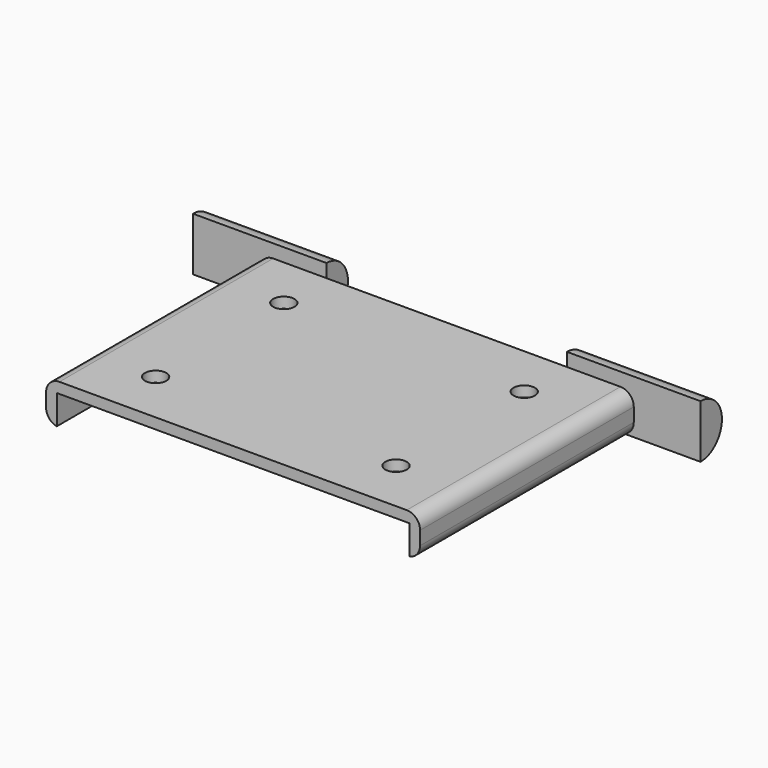
from build123d import *

# Parameters (mm, degrees)
F1_DEPTH    = 100
F2_T1_DEPTH = 125
F2_T3_DEPTH = 124.4948974279
F3_T1_DEPTH = 124.4948974279
F3_T3_DEPTH = 125
F5_D        = 8
F7_R        = 7.5
F10_DEPTH   = 25
F14_DEPTH   = 25


# Not quite as in the source:
# - a fillet or chamfer that OpenCascade refuses, or shapes differently, is made with other operations: its cross-section is extruded or revolved along the edge and cut away or added


with BuildPart() as f1:
    # F0 (on Front) → F1 (new body)
    with BuildSketch(Plane.XZ):
        Polygon((140, 0), (0, 0), (0, -15), (4, -15), (4, -4), (136, -4), (136, -15), (140, -15), align=None)
    extrude(amount=F1_DEPTH)

    # F2: fillet of radius 5 on 2 edges, made by hand

    # F2_s2 → F2_t1 (cut)
    with BuildSketch(Plane.XZ.offset(-12.5)):
        with BuildLine():
            ThreePointArc((5, 0), (1.4644660941, -1.4644660941), (0, -5))
            Line((0, -5), (0, 0))
            Line((0, 0), (5, 0))
        make_face()
    extrude(amount=F2_T1_DEPTH, mode=Mode.SUBTRACT)

    # F2_s4 → F2_t3 (cut)
    with BuildSketch(Plane.XZ.offset(-12.2474487139)):
        with BuildLine():
            ThreePointArc((136, -15), (138.8729833462, -13.2632981746), (140, -10.1010205144))
            Line((140, -10.1010205144), (140, -15))
            Line((140, -15), (136, -15))
        make_face()
    extrude(amount=F2_T3_DEPTH, mode=Mode.SUBTRACT)

    # F3: fillet of radius 5 on 2 edges, made by hand

    # F3_s2 → F3_t1 (cut)
    with BuildSketch(Plane.XZ.offset(-12.2474487139)):
        with BuildLine():
            ThreePointArc((4, -15), (1.1270166538, -13.2632981746), (0, -10.1010205144))
            Line((0, -10.1010205144), (0, -15))
            Line((0, -15), (4, -15))
        make_face()
    extrude(amount=F3_T1_DEPTH, mode=Mode.SUBTRACT)

    # F3_s4 → F3_t3 (cut)
    with BuildSketch(Plane.XZ.offset(-12.5)):
        with BuildLine():
            ThreePointArc((135, 0), (138.5355339059, -1.4644660941), (140, -5))
            Line((140, -5), (140, 0))
            Line((140, 0), (135, 0))
        make_face()
    extrude(amount=F3_T3_DEPTH, mode=Mode.SUBTRACT)

    # F5 (through all)
    with Locations(Plane.XY):
        with Locations((25, -20), (115, -20), (25, -80), (115, -80)):
            Hole(F5_D / 2)

    # F9 (on Right) → F10 (join, symmetric)
    with BuildSketch(Plane.YZ):
        with BuildLine():
            Line((0, 5), (0, 0))
            Line((0, 0), (0, -5))
            Line((0, -5), (0, -15))
            ThreePointArc((0, -15), (10, -5), (0, 5))
        make_face()
    extrude(amount=F10_DEPTH, both=True)

    # F13 (on offset) → F14 (join, symmetric)
    with BuildSketch(Plane.YZ.offset(140)):
        with BuildLine():
            Line((0, -10.1010205144), (0, -15))
            ThreePointArc((0, -15), (10, -5), (0, 5))
            Line((0, 5), (0, 0))
            Line((0, 0), (0, -5))
            Line((0, -5), (0, -10.1010205144))
        make_face()
    extrude(amount=F14_DEPTH, both=True)


with BuildPart() as f8:
    # F8: sweep along a path in F6
    with BuildLine(Plane.XZ) as f8_path:
        Line((-40, 0), (-40, 100))
        ThreePointArc((-40, 100), (-85, 150), (-130, 100))
        Line((-130, 100), (-130, 0))
    # F7 (on Top) → F8 (sweep)
    with BuildSketch(Plane.XY):
        with Locations((-40, 0)):
            Circle(F7_R)
    sweep(path=f8_path.line)


solid = f1.part
